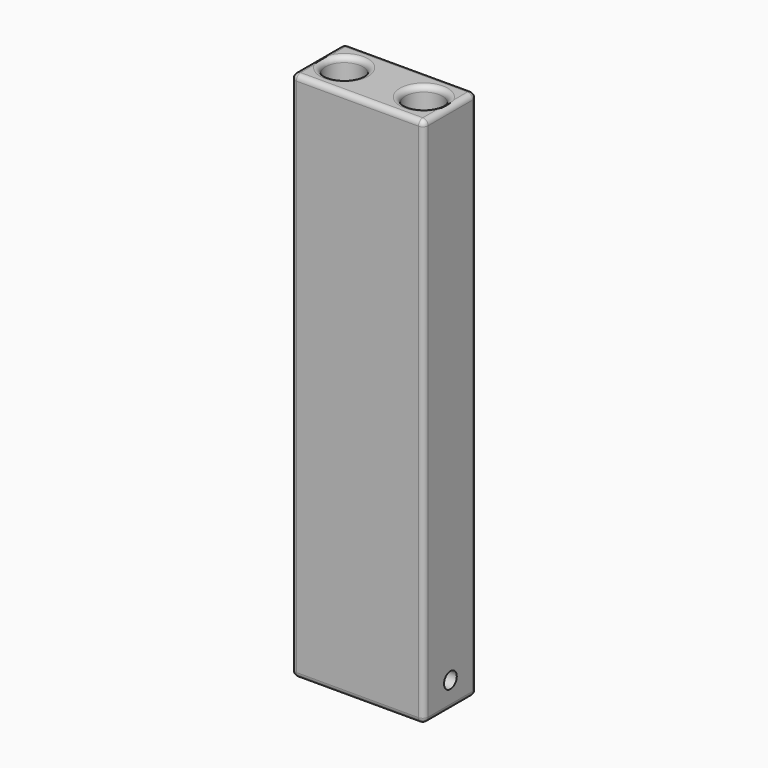
from build123d import *

# Parameters (mm, degrees)
F0_W         = 25
F0_H         = 100
F1_DEPTH     = 12.5
F2_R         = 1.5
F3_DEPTH     = 27.19003
F4_R         = 3.5
F5_DEPTH     = 10
F6_T1_DEPTH  = 10.5
F6_T3_DEPTH  = 23
F6_T5_DEPTH  = 98
F6_S9_W      = 1
F6_S9_H      = 1
F6_T10_DEPTH = 1
F6_S15_W     = 1
F6_S15_H     = 1
F6_T16_DEPTH = 1
F6_S21_W     = 1
F6_S21_H     = 1
F6_T22_DEPTH = 1
F6_S27_W     = 1
F6_S27_H     = 1
F6_T28_DEPTH = 1
F6_S33_W     = 1
F6_S33_H     = 1
F6_T34_DEPTH = 1
F6_S39_W     = 1
F6_S39_H     = 1
F6_T40_DEPTH = 1
F6_S45_W     = 1
F6_S45_H     = 1
F6_T46_DEPTH = 1
F6_S51_W     = 1
F6_S51_H     = 1
F6_T52_DEPTH = 1


# Not quite as in the source:
# - a fillet or chamfer that OpenCascade refuses, or shapes differently, is made with other operations: its cross-section is extruded or revolved along the edge and cut away or added


with BuildPart() as f1:
    # F0 (on Front) → F1 (new body)
    with BuildSketch(Plane.XZ):
        with Locations((-13.6877183104, 5.2395616682)):
            Rectangle(F0_W, F0_H)
    extrude(amount=F1_DEPTH)

    # F2 (on Right) → F3 (cut)
    with BuildSketch(Plane.YZ):
        with Locations((-6.25, -39.7604383318)):
            Circle(F2_R)
    extrude(amount=-F3_DEPTH, mode=Mode.SUBTRACT)

    # F4 (on face) → F5 (cut)
    with BuildSketch(Plane.XY.offset(55.2395616682)):
        with Locations((-6.1877183104, -6.25)):
            Circle(F4_R)
        with Locations((-21.1877183104, -6.25)):
            Circle(F4_R)
    extrude(amount=-F5_DEPTH, mode=Mode.SUBTRACT)

    # F6: fillet of radius 1 on 15 edges, made by hand

    # F6_s2 → F6_t1 (cut)
    with BuildSketch(Plane.XZ.offset(1)):
        with BuildLine():
            ThreePointArc((-25.1877183104, 55.2395616682), (-25.8948250916, 54.9466684494), (-26.1877183104, 54.2395616682))
            Line((-26.1877183104, 54.2395616682), (-26.1877183104, 55.2395616682))
            Line((-26.1877183104, 55.2395616682), (-25.1877183104, 55.2395616682))
        make_face()
        with BuildLine():
            ThreePointArc((-2.1877183104, 55.2395616682), (-1.4806115292, 54.9466684494), (-1.1877183104, 54.2395616682))
            Line((-1.1877183104, 54.2395616682), (-1.1877183104, 55.2395616682))
            Line((-1.1877183104, 55.2395616682), (-2.1877183104, 55.2395616682))
        make_face()
        with BuildLine():
            ThreePointArc((-26.1877183104, -43.7604383318), (-25.8948250916, -44.467545113), (-25.1877183104, -44.7604383318))
            Line((-25.1877183104, -44.7604383318), (-26.1877183104, -44.7604383318))
            Line((-26.1877183104, -44.7604383318), (-26.1877183104, -43.7604383318))
        make_face()
        with BuildLine():
            ThreePointArc((-1.1877183104, -43.7604383318), (-1.4806115292, -44.467545113), (-2.1877183104, -44.7604383318))
            Line((-2.1877183104, -44.7604383318), (-1.1877183104, -44.7604383318))
            Line((-1.1877183104, -44.7604383318), (-1.1877183104, -43.7604383318))
        make_face()
    extrude(amount=F6_T1_DEPTH, mode=Mode.SUBTRACT)

    # F6_s4 → F6_t3 (cut)
    with BuildSketch(Plane.YZ.offset(-25.1877183104)):
        with BuildLine():
            ThreePointArc((-11.5, 55.2395616682), (-12.2071067812, 54.9466684494), (-12.5, 54.2395616682))
            Line((-12.5, 54.2395616682), (-12.5, 55.2395616682))
            Line((-12.5, 55.2395616682), (-11.5, 55.2395616682))
        make_face()
        with BuildLine():
            ThreePointArc((-1, 55.2395616682), (-0.2928932188, 54.9466684494), (0, 54.2395616682))
            Line((0, 54.2395616682), (0, 55.2395616682))
            Line((0, 55.2395616682), (-1, 55.2395616682))
        make_face()
        with BuildLine():
            ThreePointArc((0, -43.7604383318), (-0.2928932188, -44.467545113), (-1, -44.7604383318))
            Line((-1, -44.7604383318), (0, -44.7604383318))
            Line((0, -44.7604383318), (0, -43.7604383318))
        make_face()
        with BuildLine():
            ThreePointArc((-12.5, -43.7604383318), (-12.2071067812, -44.467545113), (-11.5, -44.7604383318))
            Line((-11.5, -44.7604383318), (-12.5, -44.7604383318))
            Line((-12.5, -44.7604383318), (-12.5, -43.7604383318))
        make_face()
    extrude(amount=F6_T3_DEPTH, mode=Mode.SUBTRACT)

    # F6_s6 → F6_t5 (cut)
    with BuildSketch(Plane.XY.offset(-43.7604383318)):
        with BuildLine():
            ThreePointArc((-25.1877183104, 0), (-25.8948250916, -0.2928932188), (-26.1877183104, -1))
            Line((-26.1877183104, -1), (-26.1877183104, 0))
            Line((-26.1877183104, 0), (-25.1877183104, 0))
        make_face()
        with BuildLine():
            ThreePointArc((-1.1877183104, -1), (-1.4806115292, -0.2928932188), (-2.1877183104, 0))
            Line((-2.1877183104, 0), (-1.1877183104, 0))
            Line((-1.1877183104, 0), (-1.1877183104, -1))
        make_face()
        with BuildLine():
            ThreePointArc((-25.1877183104, -12.5), (-25.8948250916, -12.2071067812), (-26.1877183104, -11.5))
            Line((-26.1877183104, -11.5), (-26.1877183104, -12.5))
            Line((-26.1877183104, -12.5), (-25.1877183104, -12.5))
        make_face()
        with BuildLine():
            ThreePointArc((-1.1877183104, -11.5), (-1.4806115292, -12.2071067812), (-2.1877183104, -12.5))
            Line((-2.1877183104, -12.5), (-1.1877183104, -12.5))
            Line((-1.1877183104, -12.5), (-1.1877183104, -11.5))
        make_face()
    extrude(amount=F6_T5_DEPTH, mode=Mode.SUBTRACT)


with BuildPart() as f6_tool8:
    # F6_s9 → F6_t10 (new body)
    with BuildSketch(Plane.XY.offset(54.2395616682)):
        with Locations((-25.6877183104, -0.5)):
            Rectangle(F6_S9_W, F6_S9_H)
    extrude(amount=F6_T10_DEPTH)

    # F6_s11 → F6_t12 (revolve, cut)
    with BuildSketch(Plane(origin=(-25.1877183104, -1, 54.2395616682), x_dir=(0.7071067812, -0.7071067812, 0), z_dir=(-0.7071067812, -0.7071067812, 0))):
        with BuildLine():
            ThreePointArc((0, -1), (1, 0), (0, 1))
            Line((0, 1), (0, -1))
        make_face()
    revolve(axis=Axis((-25.1877183104, -1, 54.2395616682), (0, 0, 1)), mode=Mode.SUBTRACT)


with BuildPart() as f1_1:
    add(f1.part)

    # F6_t7: cut F6_tool8
    add(f6_tool8.part, mode=Mode.SUBTRACT)


with BuildPart() as f6_tool14:
    # F6_s15 → F6_t16 (new body)
    with BuildSketch(Plane.XY.offset(54.2395616682)):
        with Locations((-25.6877183104, -12)):
            Rectangle(F6_S15_W, F6_S15_H)
    extrude(amount=F6_T16_DEPTH)

    # F6_s17 → F6_t18 (revolve, cut)
    with BuildSketch(Plane(origin=(-25.1877183104, -11.5, 54.2395616682), x_dir=(0.7071067812, 0.7071067812, 0), z_dir=(0.7071067812, -0.7071067812, 0))):
        with BuildLine():
            ThreePointArc((0, -1), (1, 0), (0, 1))
            Line((0, 1), (0, -1))
        make_face()
    revolve(axis=Axis((-25.1877183104, -11.5, 54.2395616682), (0, 0, 1)), mode=Mode.SUBTRACT)


with BuildPart() as f1_2:
    add(f1_1.part)

    # F6_t13: cut F6_tool14
    add(f6_tool14.part, mode=Mode.SUBTRACT)


with BuildPart() as f6_tool20:
    # F6_s21 → F6_t22 (new body)
    with BuildSketch(Plane.XY.offset(54.2395616682)):
        with Locations((-1.6877183104, -12)):
            Rectangle(F6_S21_W, F6_S21_H)
    extrude(amount=F6_T22_DEPTH)

    # F6_s23 → F6_t24 (revolve, cut)
    with BuildSketch(Plane(origin=(-2.1877183104, -11.5, 54.2395616682), x_dir=(-0.7071067812, 0.7071067812, 0), z_dir=(0.7071067812, 0.7071067812, 0))):
        with BuildLine():
            ThreePointArc((0, -1), (1, 0), (0, 1))
            Line((0, 1), (0, -1))
        make_face()
    revolve(axis=Axis((-2.1877183104, -11.5, 54.2395616682), (0, 0, 1)), mode=Mode.SUBTRACT)


with BuildPart() as f1_3:
    add(f1_2.part)

    # F6_t19: cut F6_tool20
    add(f6_tool20.part, mode=Mode.SUBTRACT)


with BuildPart() as f6_tool26:
    # F6_s27 → F6_t28 (new body)
    with BuildSketch(Plane.XY.offset(54.2395616682)):
        with Locations((-1.6877183104, -0.5)):
            Rectangle(F6_S27_W, F6_S27_H)
    extrude(amount=F6_T28_DEPTH)

    # F6_s29 → F6_t30 (revolve, cut)
    with BuildSketch(Plane(origin=(-2.1877183104, -1, 54.2395616682), x_dir=(-0.7071067812, -0.7071067812, 0), z_dir=(-0.7071067812, 0.7071067812, 0))):
        with BuildLine():
            ThreePointArc((0, -1), (1, 0), (0, 1))
            Line((0, 1), (0, -1))
        make_face()
    revolve(axis=Axis((-2.1877183104, -1, 54.2395616682), (0, 0, 1)), mode=Mode.SUBTRACT)


with BuildPart() as f1_4:
    add(f1_3.part)

    # F6_t25: cut F6_tool26
    add(f6_tool26.part, mode=Mode.SUBTRACT)


with BuildPart() as f6_tool32:
    # F6_s33 → F6_t34 (new body)
    with BuildSketch(Plane.XZ.offset(1)):
        with Locations((-25.6877183104, -44.2604383318)):
            Rectangle(F6_S33_W, F6_S33_H)
    extrude(amount=-F6_T34_DEPTH)

    # F6_s35 → F6_t36 (revolve, cut)
    with BuildSketch(Plane(origin=(-25.1877183104, -1, -43.7604383318), x_dir=(0.7071067812, 0, 0.7071067812), z_dir=(-0.7071067812, 0, 0.7071067812))):
        with BuildLine():
            ThreePointArc((0, -1), (1, 0), (0, 1))
            Line((0, 1), (0, -1))
        make_face()
    revolve(axis=Axis((-25.1877183104, -1, -43.7604383318), (0, 1, 0)), mode=Mode.SUBTRACT)


with BuildPart() as f1_5:
    add(f1_4.part)

    # F6_t31: cut F6_tool32
    add(f6_tool32.part, mode=Mode.SUBTRACT)


with BuildPart() as f6_tool38:
    # F6_s39 → F6_t40 (new body)
    with BuildSketch(Plane.YZ.offset(-2.1877183104)):
        with Locations((-0.5, -44.2604383318)):
            Rectangle(F6_S39_W, F6_S39_H)
    extrude(amount=F6_T40_DEPTH)

    # F6_s41 → F6_t42 (revolve, cut)
    with BuildSketch(Plane(origin=(-2.1877183104, -1, -43.7604383318), x_dir=(0, -0.7071067812, 0.7071067812), z_dir=(0, 0.7071067812, 0.7071067812))):
        with BuildLine():
            ThreePointArc((0, -1), (1, 0), (0, 1))
            Line((0, 1), (0, -1))
        make_face()
    revolve(axis=Axis((-2.1877183104, -1, -43.7604383318), (1, 0, 0)), mode=Mode.SUBTRACT)


with BuildPart() as f1_6:
    add(f1_5.part)

    # F6_t37: cut F6_tool38
    add(f6_tool38.part, mode=Mode.SUBTRACT)


with BuildPart() as f6_tool44:
    # F6_s45 → F6_t46 (new body)
    with BuildSketch(Plane.XZ.offset(11.5)):
        with Locations((-25.6877183104, -44.2604383318)):
            Rectangle(F6_S45_W, F6_S45_H)
    extrude(amount=F6_T46_DEPTH)

    # F6_s47 → F6_t48 (revolve, cut)
    with BuildSketch(Plane(origin=(-25.1877183104, -11.5, -43.7604383318), x_dir=(0.7071067812, 0, 0.7071067812), z_dir=(0.7071067812, 0, -0.7071067812))):
        with BuildLine():
            ThreePointArc((0, -1), (1, 0), (0, 1))
            Line((0, 1), (0, -1))
        make_face()
    revolve(axis=Axis((-25.1877183104, -11.5, -43.7604383318), (0, -1, 0)), mode=Mode.SUBTRACT)


with BuildPart() as f1_7:
    add(f1_6.part)

    # F6_t43: cut F6_tool44
    add(f6_tool44.part, mode=Mode.SUBTRACT)


with BuildPart() as f6_tool50:
    # F6_s51 → F6_t52 (new body)
    with BuildSketch(Plane.YZ.offset(-2.1877183104)):
        with Locations((-12, -44.2604383318)):
            Rectangle(F6_S51_W, F6_S51_H)
    extrude(amount=F6_T52_DEPTH)

    # F6_s53 → F6_t54 (revolve, cut)
    with BuildSketch(Plane(origin=(-2.1877183104, -11.5, -43.7604383318), x_dir=(0, 0.7071067812, 0.7071067812), z_dir=(0, 0.7071067812, -0.7071067812))):
        with BuildLine():
            ThreePointArc((0, -1), (1, 0), (0, 1))
            Line((0, 1), (0, -1))
        make_face()
    revolve(axis=Axis((-2.1877183104, -11.5, -43.7604383318), (1, 0, 0)), mode=Mode.SUBTRACT)


with BuildPart() as f1_8:
    add(f1_7.part)

    # F6_t49: cut F6_tool50
    add(f6_tool50.part, mode=Mode.SUBTRACT)

    # F6_s55 → F6_t56 (revolve, cut)
    with BuildSketch(Plane.XY.offset(-39.7604383318)):
        with BuildLine():
            ThreePointArc((-26.1877183104, -3.75), (-25.8948250916, -4.4571067812), (-25.1877183104, -4.75))
            Line((-25.1877183104, -4.75), (-26.1877183104, -4.75))
            Line((-26.1877183104, -4.75), (-26.1877183104, -3.75))
        make_face()
    revolve(axis=Axis((-26.1877183104, -6.25, -39.7604383318), (1, 0, 0)), mode=Mode.SUBTRACT)

    # F6_s57 → F6_t58 (revolve, cut)
    with BuildSketch(Plane.XZ.offset(6.25)):
        with BuildLine():
            ThreePointArc((-16.6877183104, 55.2395616682), (-17.3948250916, 54.9466684494), (-17.6877183104, 54.2395616682))
            Line((-17.6877183104, 54.2395616682), (-17.6877183104, 55.2395616682))
            Line((-17.6877183104, 55.2395616682), (-16.6877183104, 55.2395616682))
        make_face()
    revolve(axis=Axis((-21.1877183104, -6.25, 55.2395616682), (0, 0, 1)), mode=Mode.SUBTRACT)

    # F6_s59 → F6_t60 (revolve, cut)
    with BuildSketch(Plane.XZ.offset(6.25)):
        with BuildLine():
            ThreePointArc((-1.6877183104, 55.2395616682), (-2.3948250916, 54.9466684494), (-2.6877183104, 54.2395616682))
            Line((-2.6877183104, 54.2395616682), (-2.6877183104, 55.2395616682))
            Line((-2.6877183104, 55.2395616682), (-1.6877183104, 55.2395616682))
        make_face()
    revolve(axis=Axis((-6.1877183104, -6.25, 55.2395616682), (0, 0, 1)), mode=Mode.SUBTRACT)


solid = f1_8.part
